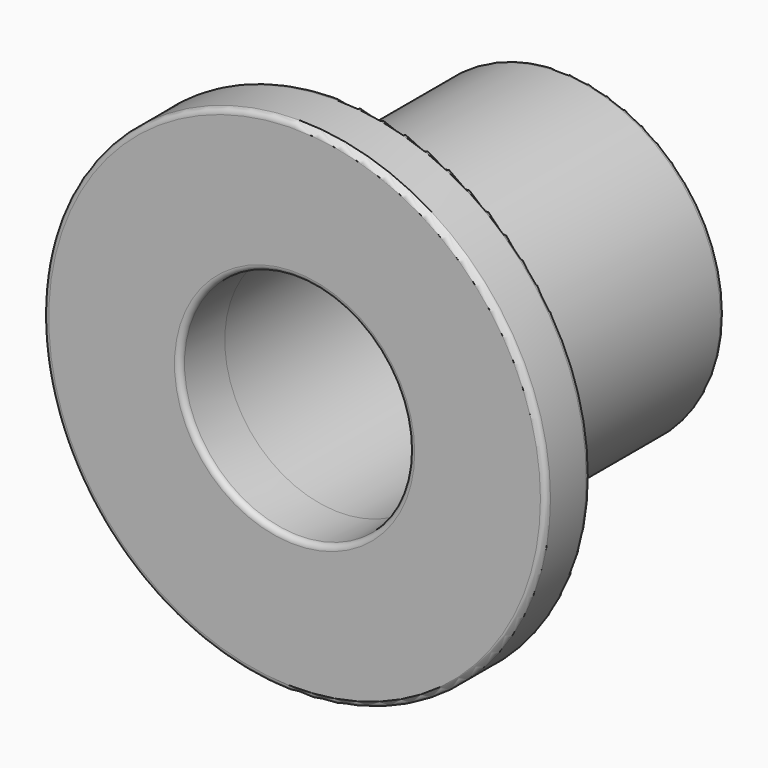
from build123d import *

# Parameters (mm, degrees)
F0_R     = 9
F0_R_2   = 5.8
F0_R_3   = 4.1
F1_DEPTH = 2
F2_DEPTH = 10
F3_R     = 0.2


# Not quite as in the source:
# - a feature names something its author has since deleted; it is built from what else it names


with BuildPart() as f1:
    # F0 (on Front) → F1 (new body)
    with BuildSketch(Plane.XZ):
        Circle(F0_R)
        Circle(F0_R_2, mode=Mode.SUBTRACT)
        Circle(F0_R_2)
        Circle(F0_R_3, mode=Mode.SUBTRACT)
    extrude(amount=F1_DEPTH)

    # F0 (on Front) → F2 (join)
    with BuildSketch(Plane.XZ):
        Circle(F0_R_2)
        Circle(F0_R_3, mode=Mode.SUBTRACT)
    extrude(amount=-F2_DEPTH)

    # F3
    f3_edges = [f1.edges().sort_by_distance(p)[0] for p in [
        (-9, 0, 0),
        (-9, -2, 0),
        (5.8, 5, 0),
        (-5.8, 0, 0),
        (-5.8, 10, 0),
        (-4.1, 10, 0),
        (-4.1, -2, 0),
    ]]
    fillet(f3_edges, radius=F3_R)


solid = f1.part
